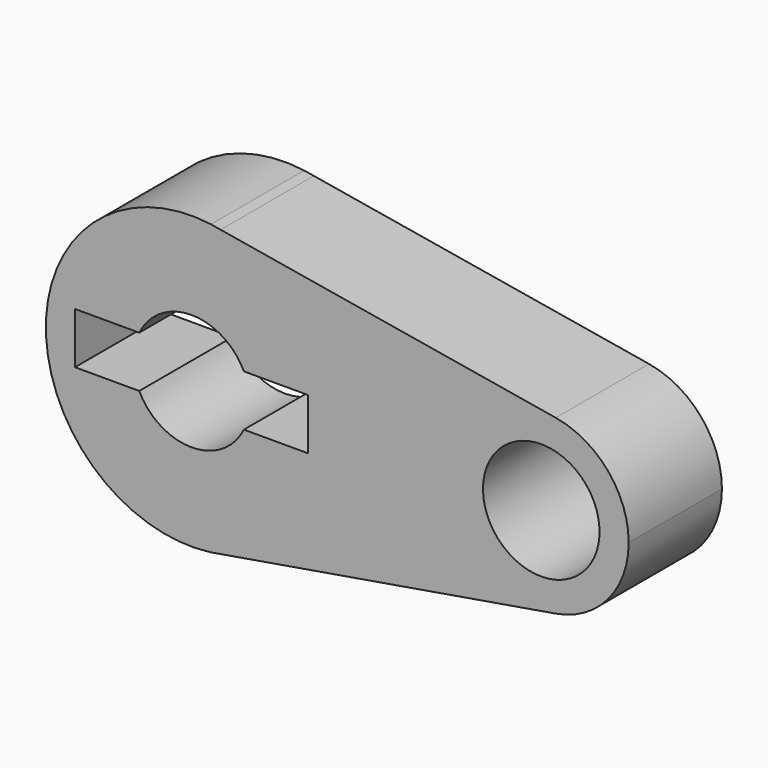
from build123d import *

# Parameters (mm, degrees)
F1_DEPTH = 25.4


with BuildPart() as f1:
    # F0 (on Front) → F1 (new body)
    with BuildSketch(Plane.XZ):
        with BuildLine():
            Line((6.3292504433, 31.1127480115), (4.2333333333, 31.4665121818))
            ThreePointArc((4.2333333333, 31.4665121818), (-31.75, 0), (4.2333333333, -31.4665121818))
            Line((4.2333333333, -31.4665121818), (6.3292504433, -31.1127480115))
            ThreePointArc((6.3292504433, -31.1127480115), (24.5867464457, -20.0886634501), (31.75, 0))
            ThreePointArc((31.75, 0), (24.5867464457, 20.0886634501), (6.3292504433, 31.1127480115))
        make_face()
        with BuildLine():
            Line((25.4, 5.588), (25.4, 0))
            Line((25.4, 0), (25.4, -5.588))
            Line((25.4, -5.588), (11.4045717149, -5.588))
            ThreePointArc((11.4045717149, -5.588), (0, -12.7), (-11.4045717149, -5.588))
            Line((-11.4045717149, -5.588), (-25.4, -5.588))
            Line((-25.4, -5.588), (-25.4, 5.588))
            Line((-25.4, 5.588), (-11.4045717149, 5.588))
            ThreePointArc((-11.4045717149, 5.588), (0, 12.7), (11.4045717149, 5.588))
            Line((11.4045717149, 5.588), (25.4, 5.588))
        make_face(mode=Mode.SUBTRACT)
        with BuildLine():
            Line((79.3705518859, 18.7843046381), (6.3292504433, 31.1127480115))
            ThreePointArc((6.3292504433, 31.1127480115), (24.5867464457, 20.0886634501), (31.75, 0))
            Line((31.75, 0), (57.15, 0))
            ThreePointArc((57.15, 0), (63.9015552493, 14.5482217715), (79.3705518859, 18.7843046381))
        make_face()
        with BuildLine():
            ThreePointArc((31.75, 0), (24.5867464457, -20.0886634501), (6.3292504433, -31.1127480115))
            Line((6.3292504433, -31.1127480115), (79.3705518859, -18.7843046381))
            ThreePointArc((79.3705518859, -18.7843046381), (63.9015552493, -14.5482217715), (57.15, 0))
            Line((57.15, 0), (31.75, 0))
        make_face()
        with BuildLine():
            ThreePointArc((95.25, 0), (90.7482217715, 12.2984447507), (79.3705518859, 18.7843046381))
            ThreePointArc((79.3705518859, 18.7843046381), (63.9015552493, 14.5482217715), (57.15, 0))
            ThreePointArc((57.15, 0), (63.9015552493, -14.5482217715), (79.3705518859, -18.7843046381))
            ThreePointArc((79.3705518859, -18.7843046381), (90.7482217715, -12.2984447507), (95.25, 0))
        make_face()
        with BuildLine():
            ThreePointArc((88.9, 0), (76.2, -12.7), (63.5, 0))
            ThreePointArc((63.5, 0), (76.2, 12.7), (88.9, 0))
        make_face(mode=Mode.SUBTRACT)
    extrude(amount=F1_DEPTH)


solid = f1.part
